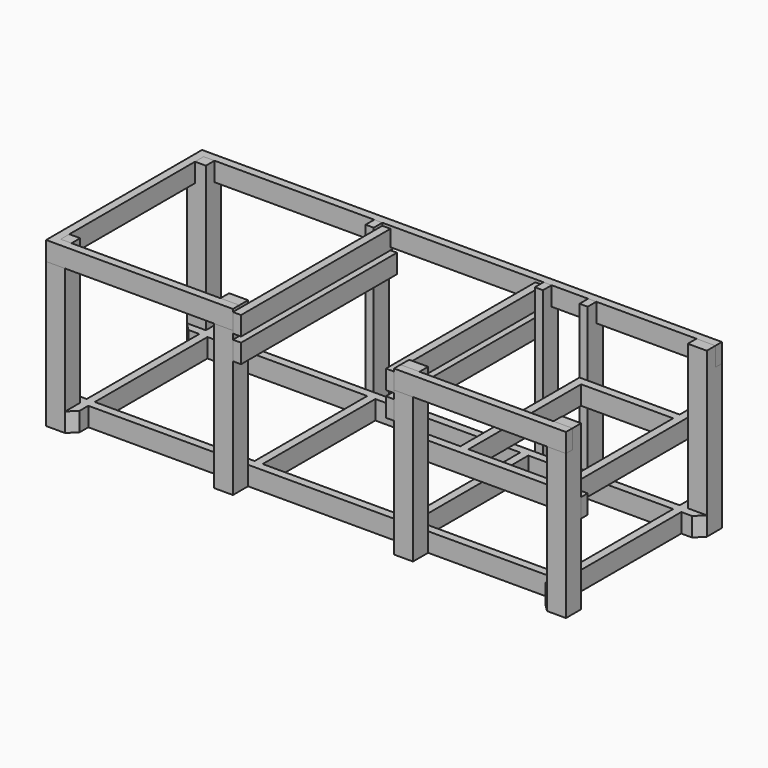
from build123d import *

# Parameters (mm, degrees)
F0_W      = 88.9
F0_H      = 88.9
F1_DEPTH  = 768.35
F2_W      = 2184.4
F2_H      = 660.4
F3_DEPTH  = 88.9
F4_SIZE   = 38.09999
F5_W      = 38.1
F5_H      = 660.4
F6_DEPTH  = 88.9
F7_W      = 38.1
F7_H      = 88.9
F8_DEPTH  = 768.35
F13_W     = 38.1
F13_H     = 660.4
F14_DEPTH = 88.9
F15_W     = 38.1
F15_H     = 914.4
F16_DEPTH = 88.9
F17_W     = 38.1
F17_H     = 914.4
F18_DEPTH = 88.9
F19_DEPTH = 88.9
F12_W     = 806.45
F12_H     = 38.1


# Not quite as in the source:
# - a fillet or chamfer is up to 0.001 mm smaller than in the source, because OpenCascade refuses the exact size


with BuildPart() as f1:
    # F0 (on Top) → F1 (new body)
    with BuildSketch(Plane.XY):
        with Locations((-1174.75, -412.75)):
            Rectangle(F0_W, F0_H)
    extrude(amount=F1_DEPTH)


with BuildPart() as f1b:
    # F0 (on Top) → F1, piece 2 (new body)
    with BuildSketch(Plane.XY):
        with Locations((-1174.75, 412.75)):
            Rectangle(F0_W, F0_H)
    extrude(amount=F1_DEPTH)


with BuildPart() as f1c:
    # F0 (on Top) → F1, piece 3 (new body)
    with BuildSketch(Plane.XY):
        with Locations((1174.75, -412.75)):
            Rectangle(F0_W, F0_H)
    extrude(amount=F1_DEPTH)


with BuildPart() as f1d:
    # F0 (on Top) → F1, piece 4 (new body)
    with BuildSketch(Plane.XY):
        with Locations((1174.75, 412.75)):
            Rectangle(F0_W, F0_H)
    extrude(amount=F1_DEPTH)


with BuildPart() as f1e:
    # F0 (on Top) → F1, piece 5 (new body)
    with BuildSketch(Plane.XY):
        with Locations((-387.35, -412.75)):
            Rectangle(F0_W, F0_H)
    extrude(amount=F1_DEPTH)


with BuildPart() as f1f:
    # F0 (on Top) → F1, piece 6 (new body)
    with BuildSketch(Plane.XY):
        with Locations((457.2, -412.75)):
            Rectangle(F0_W, F0_H)
    extrude(amount=F1_DEPTH)


with BuildPart() as f3:
    # F2 (on Top) → F3 (new body)
    with BuildSketch(Plane.XY):
        Polygon((-1130.3, 368.3), (-1219.2, 368.3), (-1219.2, 330.2), (-1130.3, 330.2), (-1130.3, -330.2), (-1219.2, -330.2), (-1219.2, -368.3), (-1130.3, -368.3), (-1130.3, -457.2), (-1092.2, -457.2), (-1092.2, -368.3), (1092.2, -368.3), (1092.2, -457.2), (1130.3, -457.2), (1130.3, -368.3), (1219.2, -368.3), (1219.2, -330.2), (1130.3, -330.2), (1130.3, 330.2), (1219.2, 330.2), (1219.2, 368.3), (1130.3, 368.3), (1130.3, 457.2), (1092.2, 457.2), (1092.2, 368.3), (-1092.2, 368.3), (-1092.2, 457.2), (-1130.3, 457.2), align=None)
        Rectangle(F2_W, F2_H, mode=Mode.SUBTRACT)
    extrude(amount=F3_DEPTH)

    # F4 (size 38.1 in the source; OpenCascade refuses exactly that, so slightly less here)
    f4_edges = [f3.edges().sort_by_distance(p)[0] for p in [
        (-1219.2, 330.2, 44.45),
        (-1219.2, -330.2, 44.45),
        (-1092.2, -457.2, 44.45),
        (1092.2, -457.2, 44.45),
        (1219.2, 330.2, 44.45),
        (1092.2, 457.2, 44.45),
        (1219.2, -330.2, 44.45),
        (-1092.2, 457.2, 44.45),
    ]]
    chamfer(f4_edges, length=F4_SIZE)

    # F5 (on Top) → F6 (join, through all)
    with BuildSketch(Plane.XY):
        with Locations((-323.85, 0)):
            Rectangle(F5_W, F5_H)
        with Locations((393.7, 0)):
            Rectangle(F5_W, F5_H)
    extrude(amount=F6_DEPTH)

    # F7 (on Top) → F8 (join, through all)
    with BuildSketch(Plane.XY):
        with Locations((-361.95, 412.75)):
            Rectangle(F7_W, F7_H)
        with Locations((431.8, 412.75)):
            Rectangle(F7_W, F7_H)
        with Locations((641.35, 412.75)):
            Rectangle(F7_W, F7_H)
    extrude(amount=F8_DEPTH)


with BuildPart() as f14:
    # F13 (on offset) → F14 (new body)
    with BuildSketch(Plane.XY.offset(463.55)):
        Polygon((622.3, -330.2), (412.75, -330.2), (412.75, -368.3), (1219.2, -368.3), (1219.2, -330.2), (1130.3, -330.2), (1092.2, -330.2), (660.4, -330.2), align=None)
        with Locations((641.35, 0)):
            Rectangle(F13_W, F13_H)
        Polygon((622.3, 368.3), (622.3, 330.2), (660.4, 330.2), (1092.2, 330.2), (1092.2, 368.3), align=None)
        Polygon((1092.2, 330.2), (1092.2, -330.2), (1130.3, -330.2), (1130.3, 457.2), (1092.2, 457.2), (1092.2, 368.3), align=None)
    extrude(amount=-F14_DEPTH)


with BuildPart() as f16:
    # F15 (on offset) → F16 (new body)
    with BuildSketch(Plane.XY.offset(641.35)):
        with Locations((-323.85, 0)):
            Rectangle(F15_W, F15_H)
    extrude(amount=-F16_DEPTH)


with BuildPart() as f16b:
    # F15 (on offset) → F16, piece 2 (new body)
    with BuildSketch(Plane.XY.offset(641.35)):
        with Locations((393.7, 0)):
            Rectangle(F15_W, F15_H)
    extrude(amount=-F16_DEPTH)


with BuildPart() as f18:
    # F17 (on offset) → F18 (new body)
    with BuildSketch(Plane.XY.offset(666.75)):
        with Locations((-323.85, 0)):
            Rectangle(F17_W, F17_H)
    extrude(amount=F18_DEPTH)


with BuildPart() as f18b:
    # F17 (on offset) → F18, piece 2 (new body)
    with BuildSketch(Plane.XY.offset(666.75)):
        with Locations((393.7, 0)):
            Rectangle(F17_W, F17_H)
    extrude(amount=F18_DEPTH)


with BuildPart() as f19:
    # F12 (on face) → F19 (new body)
    with BuildSketch(Plane.XY.offset(768.35)):
        Polygon((1219.2, 457.2), (-1219.2, 457.2), (-1219.2, 419.1), (-1219.2, -457.2), (-1181.1, -457.2), (-342.9, -457.2), (-342.9, -419.1), (-1181.1, -419.1), (-1181.1, 419.1), (1219.2, 419.1), align=None)
    extrude(amount=-F19_DEPTH)


with BuildPart() as f19b:
    # F12 (on face) → F19, piece 2 (new body)
    with BuildSketch(Plane.XY.offset(768.35)):
        with Locations((815.975, -438.15)):
            Rectangle(F12_W, F12_H)
    extrude(amount=-F19_DEPTH)


solid = Compound([f1.part, f1b.part, f1c.part, f1d.part, f1e.part, f1f.part, f3.part, f14.part, f16.part, f16b.part, f18.part, f18b.part, f19.part, f19b.part])
